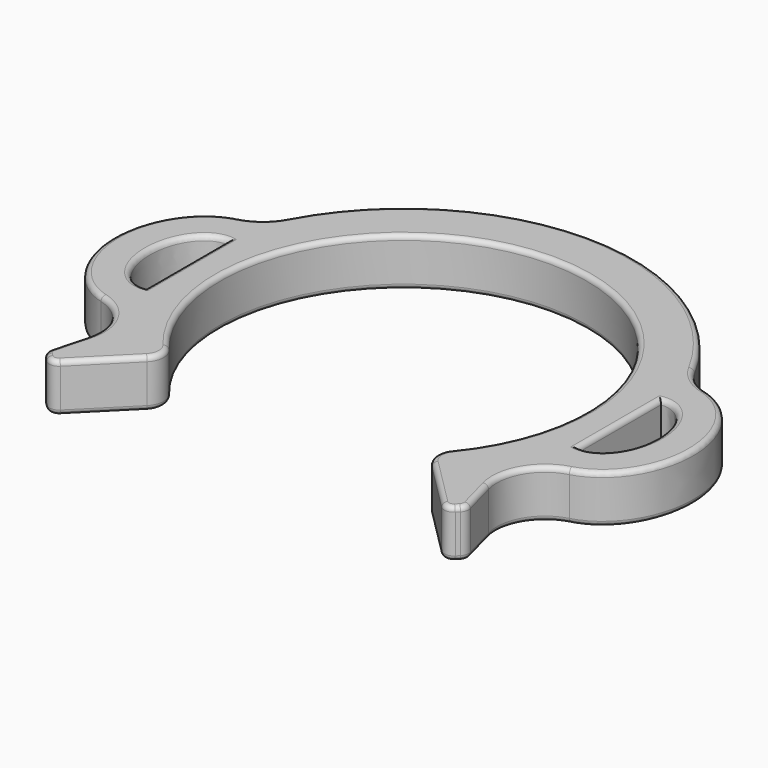
from build123d import *

# Parameters (mm, degrees)
F1_DEPTH = 5
F2_R     = 2
F3_R     = 1
F4_R     = 0.5


with BuildPart() as f1:
    # F0 (on Top) → F1 (new body)
    with BuildSketch(Plane.XY):
        with BuildLine():
            Line((-20.5414519935, -20.5414519935), (-13.4703841816, -13.4703841816))
            ThreePointArc((-13.4703841816, -13.4703841816), (0, 19.05), (13.4703841816, -13.4703841816))
            Line((13.4703841816, -13.4703841816), (20.5414519935, -20.5414519935))
            Line((20.5414519935, -20.5414519935), (21.9556655558, -19.1272384311))
            Line((21.9556655558, -19.1272384311), (20.8494967205, -14.998960136))
            ThreePointArc((20.8494967205, -14.998960136), (21.3421450158, -11.2167738297), (24.3585059831, -8.8824212185))
            add(Edge.make_bspline(
                [(24.3585059831, -8.8824212185), (30.1673484293, -7.2916773468), (30.1499684425, 0.0265760975), (30.1325884557, 7.3448295419), (24.3162895043, 8.8938231151)],
                knots=[3.3607074537, 3.3607074537, 3.3607074537, 4.7153094348, 4.7153094348, 6.0699114159, 6.0699114159, 6.0699114159], degree=2, weights=[1, 0.7792670028, 1, 0.7792670028, 1]))
            ThreePointArc((24.3162895043, 8.8938231151), (22.5001115666, 9.8047192354), (21.19631764, 11.3630373802))
            ThreePointArc((21.19631764, 11.3630373802), (12.3515474943, 20.6359340592), (0, 24.05))
            ThreePointArc((0, 24.05), (-12.3515474943, 20.6359340592), (-21.19631764, 11.3630373802))
            ThreePointArc((-21.19631764, 11.3630373802), (-22.5001115666, 9.8047192354), (-24.3162895043, 8.8938231151))
            add(Edge.make_bspline(
                [(-24.3162895043, 8.8938231151), (-30.1325884557, 7.3448295419), (-30.1499684425, 0.0265760975), (-30.1673484293, -7.2916773468), (-24.3585059831, -8.8824212185)],
                knots=[0.2132738913, 0.2132738913, 0.2132738913, 1.5678758724, 1.5678758724, 2.9224778535, 2.9224778535, 2.9224778535], degree=2, weights=[1, 0.7792670028, 1, 0.7792670028, 1]))
            ThreePointArc((-24.3585059831, -8.8824212185), (-21.3421450158, -11.2167738297), (-20.8494967205, -14.998960136))
            Line((-20.8494967205, -14.998960136), (-21.9556655558, -19.1272384311))
            Line((-21.9556655558, -19.1272384311), (-20.5414519935, -20.5414519935))
        make_face()
        with BuildLine():
            add(Edge.make_bspline(
                [(-22.5, 5.35), (-26.4, 5.7433823529), (-26.4, 0), (-26.4, -5.7433823529), (-22.5, -5.35)],
                knots=[6.2146384893, 6.2146384893, 6.2146384893, 7.853981634, 7.853981634, 9.4933247786, 9.4933247786, 9.4933247786], degree=2, weights=[1, 0.682461299, 1, 0.682461299, 1]))
            Line((-22.5, 5.35), (-22.5, -5.35))
        make_face(mode=Mode.SUBTRACT)
        with BuildLine():
            Line((22.5, -5.35), (22.5, 5.35))
            add(Edge.make_bspline(
                [(22.5, -5.35), (26.4, -5.7433823529), (26.4, 0), (26.4, 5.7433823529), (22.5, 5.35)],
                knots=[3.0730458357, 3.0730458357, 3.0730458357, 4.7123889804, 4.7123889804, 6.351732125, 6.351732125, 6.351732125], degree=2, weights=[1, 0.682461299, 1, 0.682461299, 1]))
        make_face(mode=Mode.SUBTRACT)
    extrude(amount=F1_DEPTH)

    # F2
    f2_edges = [f1.edges().sort_by_distance(p)[0] for p in [
        (-13.470384, -13.470384, 2.5),
        (13.470384, -13.470384, 2.5),
    ]]
    fillet(f2_edges, radius=F2_R)

    # F3
    f3_edges = [f1.edges().sort_by_distance(p)[0] for p in [
        (-20.541452, -20.541452, 2.5),
        (-21.955666, -19.127238, 2.5),
        (21.955666, -19.127238, 2.5),
        (20.541452, -20.541452, 2.5),
    ]]
    fillet(f3_edges, radius=F3_R)

    # F4
    f4_edges = [f1.edges().sort_by_distance(p)[0] for p in [
        (-17.325804, -17.325804, 0),
        (-20.541452, -20.127238, 0),
        (-14.233739, -13.498168, 0),
        (-21.397988, -19.684916, 0),
        (0, 19.05, 0),
        (-21.806236, -19.087199, 0),
        (14.233739, -13.498168, 0),
        (-21.327867, -16.784261, 0),
        (17.325804, -17.325804, 0),
        (-21.342145, -11.216774, 0),
        (20.541452, -20.127238, 0),
        (-30.149979, 0.021865, 0),
        (21.397988, -19.684916, 0),
        (-22.500112, 9.804719, 0),
        (21.806236, -19.087199, 0),
        (0, 24.05, 0),
        (21.327867, -16.784261, 0),
        (22.500112, 9.804719, 0),
        (21.342145, -11.216774, 0),
        (30.149979, 0.021865, 0),
        (-26.4, 0, 0),
        (-22.5, 0, 0),
        (22.5, 0, 0),
        (26.4, 0, 0),
        (-17.325804, -17.325804, 5),
        (-20.541452, -20.127238, 5),
        (-14.233739, -13.498168, 5),
        (-21.397988, -19.684916, 5),
        (0, 19.05, 5),
        (-21.806236, -19.087199, 5),
        (14.233739, -13.498168, 5),
        (-21.327867, -16.784261, 5),
        (17.325804, -17.325804, 5),
        (-21.342145, -11.216774, 5),
        (20.541452, -20.127238, 5),
        (-30.149979, 0.021865, 5),
        (21.397988, -19.684916, 5),
        (-22.500112, 9.804719, 5),
        (21.806236, -19.087199, 5),
        (0, 24.05, 5),
        (21.327867, -16.784261, 5),
        (22.500112, 9.804719, 5),
        (21.342145, -11.216774, 5),
        (30.149979, 0.021865, 5),
        (-26.4, 0, 5),
        (-22.5, 0, 5),
        (22.5, 0, 5),
        (26.4, 0, 5),
    ]]
    fillet(f4_edges, radius=F4_R)


solid = f1.part
